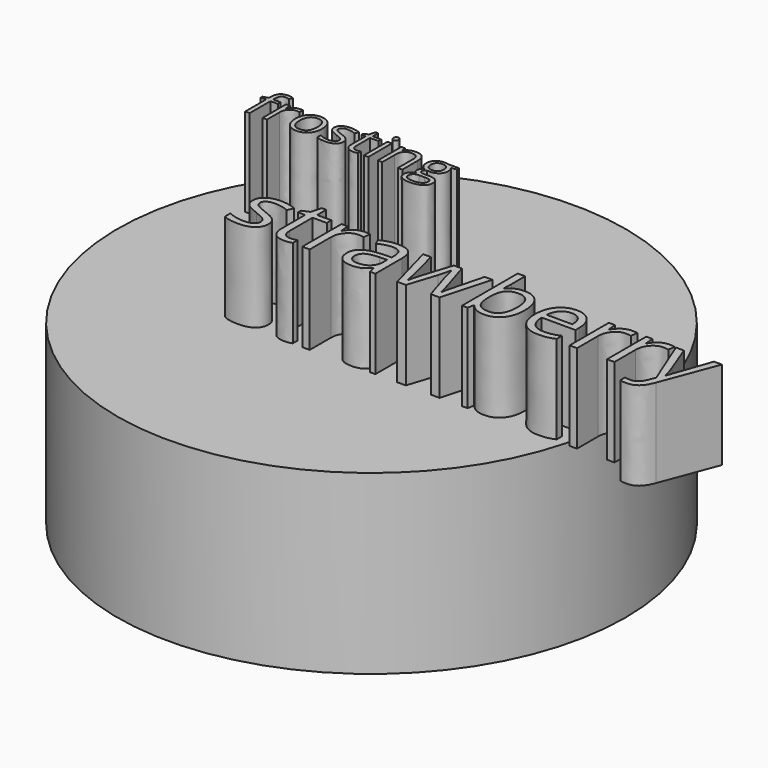
from build123d import *

# Parameters (mm, degrees)
F0_R         = 72.9508893379
F1_DEPTH     = 25.4
F2_DEPTH     = 25.4
F3_TEXT_SIZE = 26.3180118054
F4_DEPTH     = 25.4
F5_TEXT_SIZE = 15.7915159232
F6_DEPTH     = 25.4


# Not quite as in the source:
# - Text() gives the source's letters only with a copy of the font that has no kerning and outlines rounded to 1/6400 em; it was checked with that copy


with BuildPart() as f1:
    # F0 (on Top) → F1 (new body)
    with BuildSketch(Plane.XY):
        Circle(F0_R)
    extrude(amount=-F1_DEPTH)

    # F2 (add): a face of the model
    f2_faces = [f1.faces().sort_by_distance(p)[0] for p in [
        (0, 0, -25.4),
    ]]
    extrude(f2_faces, amount=F2_DEPTH)

    # F3 (on Top) → F4 (join)
    with BuildSketch(Plane.XY):
        with Locations((-28.8068397082, -18.9489684999)):
            Text('strawberry', F3_TEXT_SIZE, font='Open Sans', text_align=(TextAlign.LEFT, TextAlign.BOTTOM))
    extrude(amount=F4_DEPTH)

    # F5 (on face) → F6 (join)
    with BuildSketch(Plane.XY):
        with Locations((-57.4293020489, 24.308398366)):
            Text('frosting', F5_TEXT_SIZE, font='Open Sans', text_align=(TextAlign.LEFT, TextAlign.BOTTOM))
    extrude(amount=F6_DEPTH)


solid = f1.part
